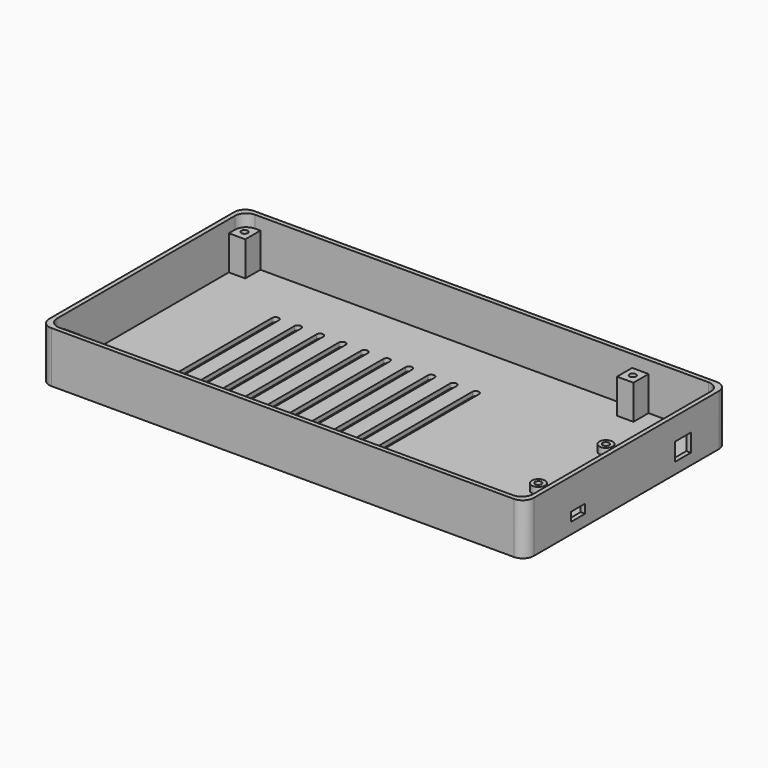
from build123d import *

# Parameters (mm, degrees)
F0_W      = 218
F0_H      = 114
F0_R      = 3
F0_R_2    = 1.75
F0_W_2    = 168.2765804879
F0_H_2    = 4.25
F0_W_3    = 167.2
F0_W_4    = 3.7
F0_H_3    = 93
F0_R_3    = 1.45
F1_DEPTH  = 2
F2_DEPTH  = 5
F3_DEPTH  = 23
F4_DEPTH  = 17.5
F7_W      = 8
F7_H      = 4
F7_W_2    = 8.9433642089
F7_H_2    = 8
F8_DEPTH  = 2
F9_R      = 5
F9_2_R    = 5
F10_R     = 5
F12_DEPTH = 2


# Not quite as in the source:
# - a feature of the source that left no trace in its solid (it failed there, or was rolled back) is left out


with BuildPart() as f1:
    # F0 (on Top) → F1 (new body)
    with BuildSketch(Plane.XY):
        with Locations((16, 0)):
            Rectangle(F0_W, F0_H)
        Polygon((84.6765804879, -55), (-83.6, -55), (-91, -55), (-91, -46.5), (-91, 46.5), (-91, 55), (-83.6, 55), (83.6, 55), (91, 55), (123, 55), (123, -55), (91, -55), (89.9765804879, -55), align=None, mode=Mode.SUBTRACT)
        with BuildLine():
            Line((-83.6, -46.5), (-83.6, -50.75))
            Line((-83.6, -50.75), (84.6765804879, -50.75))
            ThreePointArc((84.6765804879, -50.75), (85.4449622731, -48.8949622731), (87.3, -48.1265804879))
            Line((87.3, -48.1265804879), (87.3, 46.5))
            Line((87.3, 46.5), (83.6, 46.5))
            Line((83.6, 46.5), (83.6, 50.75))
            Line((83.6, 50.75), (-83.6, 50.75))
            Line((-83.6, 50.75), (-83.6, 46.5))
            Line((-83.6, 46.5), (-87.3, 46.5))
            Line((-87.3, 46.5), (-87.3, -46.5))
            Line((-87.3, -46.5), (-83.6, -46.5))
        make_face()
        with BuildLine():
            ThreePointArc((87.3, -48.1265804879), (89.1550377269, -48.8949622731), (89.9234195121, -50.75))
            Line((89.9234195121, -50.75), (89.9765804879, -50.75))
            Line((89.9765804879, -50.75), (89.9765804879, -55))
            Line((89.9765804879, -55), (91, -55))
            Line((91, -55), (123, -55))
            Line((123, -55), (123, 55))
            Line((123, 55), (91, 55))
            Line((91, 55), (91, 46.5))
            Line((91, 46.5), (87.3, 46.5))
            Line((87.3, 46.5), (87.3, -48.1265804879))
        make_face()
        with Locations((97.6, -15.2)):
            Circle(F0_R, mode=Mode.SUBTRACT)
        with Locations((101, -27.2)):
            Circle(F0_R_2, mode=Mode.SUBTRACT)
        with Locations((117, -8.2)):
            Circle(F0_R_2, mode=Mode.SUBTRACT)
        with Locations((97.6, 22.8)):
            Circle(F0_R, mode=Mode.SUBTRACT)
        with Locations((0.538290244, -52.875)):
            Rectangle(F0_W_2, F0_H_2)
        with Locations((0, 52.875)):
            Rectangle(F0_W_3, F0_H_2)
        with Locations((-89.15, 0)):
            Rectangle(F0_W_4, F0_H_3)
        with BuildLine():
            Line((-83.6, -50.75), (-85.85, -50.75))
            ThreePointArc((-85.85, -50.75), (-88.3253048327, -51.7753048327), (-87.3, -49.3))
            Line((-87.3, -49.3), (-87.3, -46.5))
            Line((-87.3, -46.5), (-91, -46.5))
            Line((-91, -46.5), (-91, -55))
            Line((-91, -55), (-83.6, -55))
            Line((-83.6, -55), (-83.6, -50.75))
        make_face()
        with BuildLine():
            Line((87.3, 49.3), (87.3, 46.5))
            Line((87.3, 46.5), (91, 46.5))
            Line((91, 46.5), (91, 55))
            Line((91, 55), (83.6, 55))
            Line((83.6, 55), (83.6, 50.75))
            Line((83.6, 50.75), (85.85, 50.75))
            ThreePointArc((85.85, 50.75), (87.3, 52.2), (88.75, 50.75))
            ThreePointArc((88.75, 50.75), (88.3253048327, 49.7246951673), (87.3, 49.3))
        make_face()
        with BuildLine():
            Line((-91, 46.5), (-87.3, 46.5))
            Line((-87.3, 46.5), (-87.3, 49.3))
            ThreePointArc((-87.3, 49.3), (-88.3253048327, 51.7753048327), (-85.85, 50.75))
            Line((-85.85, 50.75), (-83.6, 50.75))
            Line((-83.6, 50.75), (-83.6, 55))
            Line((-83.6, 55), (-91, 55))
            Line((-91, 55), (-91, 46.5))
        make_face()
        with Locations((97.6, -15.2)):
            Circle(F0_R)
        with Locations((97.6, -15.2)):
            Circle(F0_R_3, mode=Mode.SUBTRACT)
        with Locations((97.6, 22.8)):
            Circle(F0_R)
        with Locations((97.6, 22.8)):
            Circle(F0_R_3, mode=Mode.SUBTRACT)
        with BuildLine():
            ThreePointArc((-87.3, -49.3), (-86.2746951673, -49.7246951673), (-85.85, -50.75))
            Line((-85.85, -50.75), (-83.6, -50.75))
            Line((-83.6, -50.75), (-83.6, -46.5))
            Line((-83.6, -46.5), (-87.3, -46.5))
            Line((-87.3, -46.5), (-87.3, -49.3))
        make_face()
        with BuildLine():
            Line((-87.3, 49.3), (-87.3, 46.5))
            Line((-87.3, 46.5), (-83.6, 46.5))
            Line((-83.6, 46.5), (-83.6, 50.75))
            Line((-83.6, 50.75), (-85.85, 50.75))
            ThreePointArc((-85.85, 50.75), (-86.2746951673, 49.7246951673), (-87.3, 49.3))
        make_face()
        with BuildLine():
            Line((83.6, 46.5), (87.3, 46.5))
            Line((87.3, 46.5), (87.3, 49.3))
            ThreePointArc((87.3, 49.3), (86.2746951673, 49.7246951673), (85.85, 50.75))
            Line((85.85, 50.75), (83.6, 50.75))
            Line((83.6, 50.75), (83.6, 46.5))
        make_face()
        with BuildLine():
            ThreePointArc((89.9234195121, -50.75), (87.3, -53.3734195121), (84.6765804879, -50.75))
            Line((84.6765804879, -50.75), (84.6765804879, -55))
            Line((84.6765804879, -55), (89.9765804879, -55))
            Line((89.9765804879, -55), (89.9765804879, -50.75))
            Line((89.9765804879, -50.75), (89.9234195121, -50.75))
        make_face()
        with Locations((117, -8.2)):
            Circle(F0_R_2)
        with Locations((101, -27.2)):
            Circle(F0_R_2)
        with BuildLine():
            Line((85.85, -50.75), (84.6765804879, -50.75))
            ThreePointArc((84.6765804879, -50.75), (87.3, -53.3734195121), (89.9234195121, -50.75))
            Line((89.9234195121, -50.75), (88.75, -50.75))
            ThreePointArc((88.75, -50.75), (87.3, -52.2), (85.85, -50.75))
        make_face()
        with Locations((97.6, -15.2)):
            Circle(F0_R_3)
        with Locations((97.6, 22.8)):
            Circle(F0_R_3)
        with BuildLine():
            ThreePointArc((-87.3, -49.3), (-88.3253048327, -51.7753048327), (-85.85, -50.75))
            Line((-85.85, -50.75), (-87.3, -50.75))
            Line((-87.3, -50.75), (-87.3, -49.3))
        make_face()
        with BuildLine():
            Line((87.3, 50.75), (87.3, 49.3))
            ThreePointArc((87.3, 49.3), (88.3253048327, 49.7246951673), (88.75, 50.75))
            ThreePointArc((88.75, 50.75), (87.3, 52.2), (85.85, 50.75))
            Line((85.85, 50.75), (87.3, 50.75))
        make_face()
        with BuildLine():
            ThreePointArc((-85.85, 50.75), (-88.3253048327, 51.7753048327), (-87.3, 49.3))
            Line((-87.3, 49.3), (-87.3, 50.75))
            Line((-87.3, 50.75), (-85.85, 50.75))
        make_face()
        with BuildLine():
            ThreePointArc((87.3, -48.1265804879), (85.4449622731, -48.8949622731), (84.6765804879, -50.75))
            Line((84.6765804879, -50.75), (85.85, -50.75))
            ThreePointArc((85.85, -50.75), (86.2746951673, -49.7246951673), (87.3, -49.3))
            Line((87.3, -49.3), (87.3, -48.1265804879))
        make_face()
        with BuildLine():
            Line((88.75, -50.75), (89.9234195121, -50.75))
            ThreePointArc((89.9234195121, -50.75), (89.1550377269, -48.8949622731), (87.3, -48.1265804879))
            Line((87.3, -48.1265804879), (87.3, -49.3))
            ThreePointArc((87.3, -49.3), (88.3253048327, -49.7246951673), (88.75, -50.75))
        make_face()
        with BuildLine():
            Line((87.3, -50.75), (85.85, -50.75))
            ThreePointArc((85.85, -50.75), (87.3, -52.2), (88.75, -50.75))
            Line((88.75, -50.75), (87.3, -50.75))
        make_face()
        with BuildLine():
            Line((-87.3, -50.75), (-85.85, -50.75))
            ThreePointArc((-85.85, -50.75), (-86.2746951673, -49.7246951673), (-87.3, -49.3))
            Line((-87.3, -49.3), (-87.3, -50.75))
        make_face()
        with BuildLine():
            Line((-87.3, 50.75), (-87.3, 49.3))
            ThreePointArc((-87.3, 49.3), (-86.2746951673, 49.7246951673), (-85.85, 50.75))
            Line((-85.85, 50.75), (-87.3, 50.75))
        make_face()
        with BuildLine():
            ThreePointArc((85.85, 50.75), (86.2746951673, 49.7246951673), (87.3, 49.3))
            Line((87.3, 49.3), (87.3, 50.75))
            Line((87.3, 50.75), (85.85, 50.75))
        make_face()
        with BuildLine():
            ThreePointArc((87.3, -49.3), (86.2746951673, -49.7246951673), (85.85, -50.75))
            Line((85.85, -50.75), (87.3, -50.75))
            Line((87.3, -50.75), (87.3, -49.3))
        make_face()
        with BuildLine():
            Line((87.3, -49.3), (87.3, -50.75))
            Line((87.3, -50.75), (88.75, -50.75))
            ThreePointArc((88.75, -50.75), (88.3253048327, -49.7246951673), (87.3, -49.3))
        make_face()
    extrude(amount=F1_DEPTH)

    # F0 (on Top) → F2 (join)
    with BuildSketch(Plane.XY):
        with Locations((97.6, 22.8)):
            Circle(F0_R)
        with Locations((97.6, 22.8)):
            Circle(F0_R_3, mode=Mode.SUBTRACT)
        with Locations((97.6, -15.2)):
            Circle(F0_R)
        with Locations((97.6, -15.2)):
            Circle(F0_R_3, mode=Mode.SUBTRACT)
    extrude(amount=F2_DEPTH)

    # F9
    f9_edges = [f1.edges().sort_by_distance(p)[0] for p in [
        (-93, -57, 1),
        (-93, 57, 1),
        (125, 57, 1),
        (125, -57, 1),
    ]]
    fillet(f9_edges, radius=F9_R)

    # F11 (on face) → F12 (cut, through all)
    with BuildSketch(Plane.XY.offset(2)):
        with BuildLine():
            ThreePointArc((-54.5, 29), (-56, 30.5), (-57.5, 29))
            Line((-57.5, 29), (-57.5, -31))
            ThreePointArc((-57.5, -31), (-56, -32.5), (-54.5, -31))
            Line((-54.5, -31), (-54.5, 29))
        make_face()
        with BuildLine():
            Line((-44.5, -31), (-44.5, 29))
            ThreePointArc((-44.5, 29), (-46, 30.5), (-47.5, 29))
            Line((-47.5, 29), (-47.5, -31))
            ThreePointArc((-47.5, -31), (-46, -32.5), (-44.5, -31))
        make_face()
        with BuildLine():
            Line((-34.5, -31), (-34.5, 29))
            ThreePointArc((-34.5, 29), (-36, 30.5), (-37.5, 29))
            Line((-37.5, 29), (-37.5, -31))
            ThreePointArc((-37.5, -31), (-36, -32.5), (-34.5, -31))
        make_face()
        with BuildLine():
            Line((-24.5, -31), (-24.5, 29))
            ThreePointArc((-24.5, 29), (-26, 30.5), (-27.5, 29))
            Line((-27.5, 29), (-27.5, -31))
            ThreePointArc((-27.5, -31), (-26, -32.5), (-24.5, -31))
        make_face()
        with BuildLine():
            Line((-14.5, -31), (-14.5, 29))
            ThreePointArc((-14.5, 29), (-16, 30.5), (-17.5, 29))
            Line((-17.5, 29), (-17.5, -31))
            ThreePointArc((-17.5, -31), (-16, -32.5), (-14.5, -31))
        make_face()
        with BuildLine():
            Line((-4.5, -31), (-4.5, 29))
            ThreePointArc((-4.5, 29), (-6, 30.5), (-7.5, 29))
            Line((-7.5, 29), (-7.5, -31))
            ThreePointArc((-7.5, -31), (-6, -32.5), (-4.5, -31))
        make_face()
        with BuildLine():
            Line((5.5, -31), (5.5, 29))
            ThreePointArc((5.5, 29), (4, 30.5), (2.5, 29))
            Line((2.5, 29), (2.5, -31))
            ThreePointArc((2.5, -31), (4, -32.5), (5.5, -31))
        make_face()
        with BuildLine():
            Line((15.5, -31), (15.5, 29))
            ThreePointArc((15.5, 29), (14, 30.5), (12.5, 29))
            Line((12.5, 29), (12.5, -31))
            ThreePointArc((12.5, -31), (14, -32.5), (15.5, -31))
        make_face()
        with BuildLine():
            Line((25.5, -31), (25.5, 29))
            ThreePointArc((25.5, 29), (24, 30.5), (22.5, 29))
            Line((22.5, 29), (22.5, -31))
            ThreePointArc((22.5, -31), (24, -32.5), (25.5, -31))
        make_face()
        with BuildLine():
            Line((35.5, -31), (35.5, 29))
            ThreePointArc((35.5, 29), (34, 30.5), (32.5, 29))
            Line((32.5, 29), (32.5, -31))
            ThreePointArc((32.5, -31), (34, -32.5), (35.5, -31))
        make_face()
    extrude(amount=-F12_DEPTH, mode=Mode.SUBTRACT)


with BuildPart() as f3:
    # F0 (on Top) → F3 (new body)
    with BuildSketch(Plane.XY):
        with Locations((16, 0)):
            Rectangle(F0_W, F0_H)
        Polygon((84.6765804879, -55), (-83.6, -55), (-91, -55), (-91, -46.5), (-91, 46.5), (-91, 55), (-83.6, 55), (83.6, 55), (91, 55), (123, 55), (123, -55), (91, -55), (89.9765804879, -55), align=None, mode=Mode.SUBTRACT)
    extrude(amount=F3_DEPTH)

    # F0 (on Top) → F4 (join)
    with BuildSketch(Plane.XY):
        with BuildLine():
            Line((-87.3, 49.3), (-87.3, 46.5))
            Line((-87.3, 46.5), (-83.6, 46.5))
            Line((-83.6, 46.5), (-83.6, 50.75))
            Line((-83.6, 50.75), (-85.85, 50.75))
            ThreePointArc((-85.85, 50.75), (-86.2746951673, 49.7246951673), (-87.3, 49.3))
        make_face()
        with BuildLine():
            Line((-91, 46.5), (-87.3, 46.5))
            Line((-87.3, 46.5), (-87.3, 49.3))
            ThreePointArc((-87.3, 49.3), (-88.3253048327, 51.7753048327), (-85.85, 50.75))
            Line((-85.85, 50.75), (-83.6, 50.75))
            Line((-83.6, 50.75), (-83.6, 55))
            Line((-83.6, 55), (-91, 55))
            Line((-91, 55), (-91, 46.5))
        make_face()
        with BuildLine():
            Line((-83.6, -50.75), (-85.85, -50.75))
            ThreePointArc((-85.85, -50.75), (-88.3253048327, -51.7753048327), (-87.3, -49.3))
            Line((-87.3, -49.3), (-87.3, -46.5))
            Line((-87.3, -46.5), (-91, -46.5))
            Line((-91, -46.5), (-91, -55))
            Line((-91, -55), (-83.6, -55))
            Line((-83.6, -55), (-83.6, -50.75))
        make_face()
        with BuildLine():
            ThreePointArc((-87.3, -49.3), (-86.2746951673, -49.7246951673), (-85.85, -50.75))
            Line((-85.85, -50.75), (-83.6, -50.75))
            Line((-83.6, -50.75), (-83.6, -46.5))
            Line((-83.6, -46.5), (-87.3, -46.5))
            Line((-87.3, -46.5), (-87.3, -49.3))
        make_face()
        with BuildLine():
            ThreePointArc((-87.3, -49.3), (-88.3253048327, -51.7753048327), (-85.85, -50.75))
            Line((-85.85, -50.75), (-87.3, -50.75))
            Line((-87.3, -50.75), (-87.3, -49.3))
        make_face()
        with BuildLine():
            Line((-87.3, -50.75), (-85.85, -50.75))
            ThreePointArc((-85.85, -50.75), (-86.2746951673, -49.7246951673), (-87.3, -49.3))
            Line((-87.3, -49.3), (-87.3, -50.75))
        make_face()
        with BuildLine():
            Line((87.3, 49.3), (87.3, 46.5))
            Line((87.3, 46.5), (91, 46.5))
            Line((91, 46.5), (91, 55))
            Line((91, 55), (83.6, 55))
            Line((83.6, 55), (83.6, 50.75))
            Line((83.6, 50.75), (85.85, 50.75))
            ThreePointArc((85.85, 50.75), (87.3, 52.2), (88.75, 50.75))
            ThreePointArc((88.75, 50.75), (88.3253048327, 49.7246951673), (87.3, 49.3))
        make_face()
        with BuildLine():
            Line((83.6, 46.5), (87.3, 46.5))
            Line((87.3, 46.5), (87.3, 49.3))
            ThreePointArc((87.3, 49.3), (86.2746951673, 49.7246951673), (85.85, 50.75))
            Line((85.85, 50.75), (83.6, 50.75))
            Line((83.6, 50.75), (83.6, 46.5))
        make_face()
        with BuildLine():
            ThreePointArc((87.3, -48.1265804879), (85.4449622731, -48.8949622731), (84.6765804879, -50.75))
            Line((84.6765804879, -50.75), (85.85, -50.75))
            ThreePointArc((85.85, -50.75), (86.2746951673, -49.7246951673), (87.3, -49.3))
            Line((87.3, -49.3), (87.3, -48.1265804879))
        make_face()
        with BuildLine():
            Line((88.75, -50.75), (89.9234195121, -50.75))
            ThreePointArc((89.9234195121, -50.75), (89.1550377269, -48.8949622731), (87.3, -48.1265804879))
            Line((87.3, -48.1265804879), (87.3, -49.3))
            ThreePointArc((87.3, -49.3), (88.3253048327, -49.7246951673), (88.75, -50.75))
        make_face()
        with BuildLine():
            Line((85.85, -50.75), (84.6765804879, -50.75))
            ThreePointArc((84.6765804879, -50.75), (87.3, -53.3734195121), (89.9234195121, -50.75))
            Line((89.9234195121, -50.75), (88.75, -50.75))
            ThreePointArc((88.75, -50.75), (87.3, -52.2), (85.85, -50.75))
        make_face()
        with BuildLine():
            ThreePointArc((89.9234195121, -50.75), (87.3, -53.3734195121), (84.6765804879, -50.75))
            Line((84.6765804879, -50.75), (84.6765804879, -55))
            Line((84.6765804879, -55), (89.9765804879, -55))
            Line((89.9765804879, -55), (89.9765804879, -50.75))
            Line((89.9765804879, -50.75), (89.9234195121, -50.75))
        make_face()
    extrude(amount=F4_DEPTH)

    # F7 (on face) → F8 (cut, through all)
    with BuildSketch(Plane.YZ.offset(125)):
        with Locations((-27.2, 7)):
            Rectangle(F7_W, F7_H)
        with Locations((31.7716821045, 9)):
            Rectangle(F7_W_2, F7_H_2)
    extrude(amount=-F8_DEPTH, mode=Mode.SUBTRACT)

    # F9#2
    f9_2_edges = [f3.edges().sort_by_distance(p)[0] for p in [
        (-93, -57, 11.5),
        (-93, 57, 11.5),
        (125, 57, 11.5),
        (125, -57, 11.5),
    ]]
    fillet(f9_2_edges, radius=F9_2_R)

    # F10
    f10_edges = [f3.edges().sort_by_distance(p)[0] for p in [
        (-91, 55, 20.25),
        (123, 55, 11.5),
        (123, -55, 11.5),
        (-91, -55, 20.25),
    ]]
    fillet(f10_edges, radius=F10_R)


solid = Compound([f1.part, f3.part])
